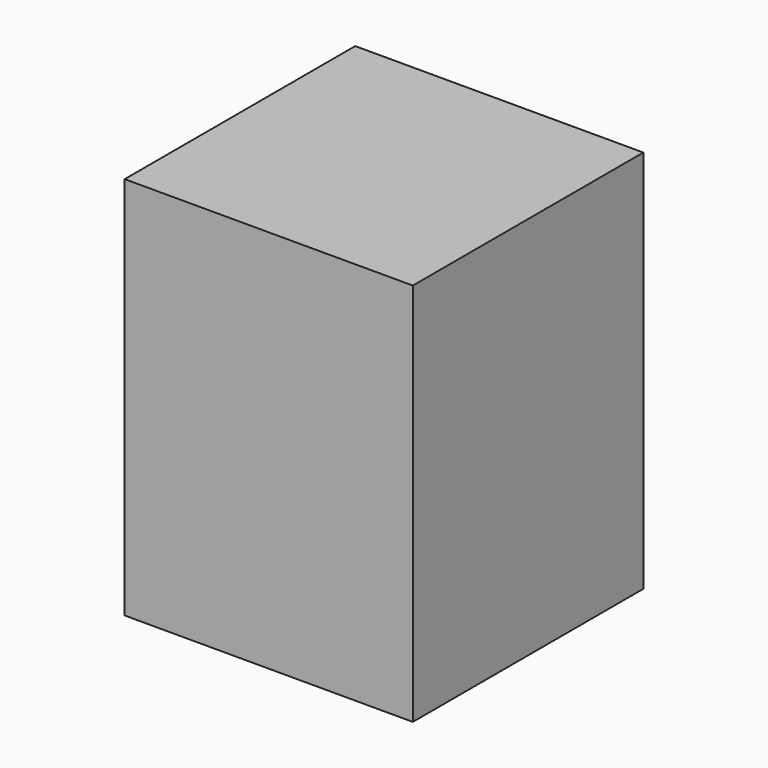
from build123d import *

# Parameters (mm, degrees)
F0_W     = 76.2
F0_H     = 101.6
F1_DEPTH = 38.1


# Not quite as in the source:
# - the program builds the solid bodies; features that only make, move or delete a surface that nothing else refers to are left out


with BuildPart() as f1:
    # F0 (on Front) → F1 (new body, symmetric)
    with BuildSketch(Plane.XZ):
        with Locations((0, 20.8269432055)):
            Rectangle(F0_W, F0_H)
    extrude(amount=F1_DEPTH, both=True)


solid = f1.part
